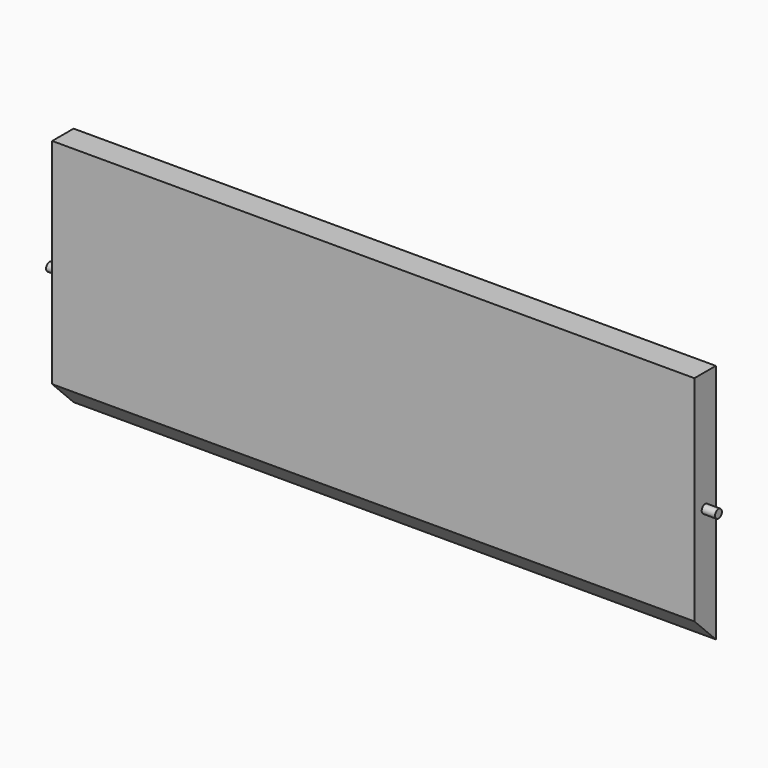
from build123d import *

# Parameters (mm, degrees)
F0_W     = 5
F0_H     = 45
F1_DEPTH = 120
F2_SIZE  = 4.99999
F3_R     = 0.8
F4_DEPTH = 2.5
F5_R     = 0.8
F6_DEPTH = 2.5


# Not quite as in the source:
# - a fillet or chamfer is up to 0.001 mm smaller than in the source, because OpenCascade refuses the exact size


with BuildPart() as f1:
    # F0 (on Right) → F1 (new body)
    with BuildSketch(Plane.YZ):
        Rectangle(F0_W, F0_H)
    extrude(amount=F1_DEPTH)

    # F2 (size 5 in the source; OpenCascade refuses exactly that, so slightly less here)
    f2_edges = [f1.edges().sort_by_distance(p)[0] for p in [
        (60, -2.5, -22.5),
    ]]
    chamfer(f2_edges, length=F2_SIZE)

    # F3 (on face) → F4 (join)
    with BuildSketch(Plane(origin=(0, 0, 0), x_dir=(0, -1, 0), z_dir=(-1, 0, 0))):
        Circle(F3_R)
    extrude(amount=F4_DEPTH)

    # F5 (on face) → F6 (join)
    with BuildSketch(Plane.YZ.offset(120)):
        Circle(F5_R)
    extrude(amount=F6_DEPTH)


solid = f1.part
